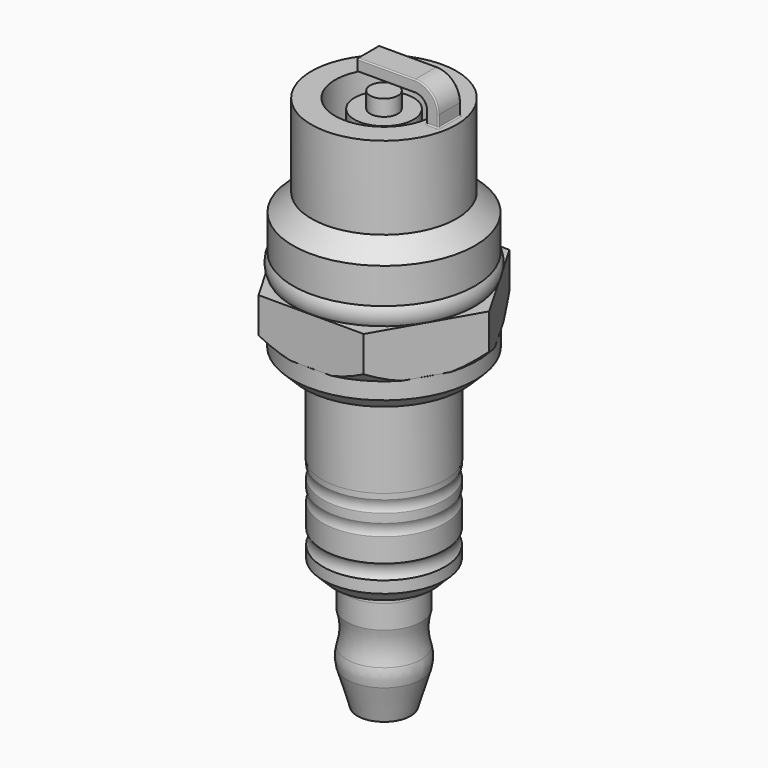
from build123d import *

# Parameters (mm, degrees)
F3_DEPTH  = 4
F4_R      = 2.5
F4_R_2    = 1.175
F5_DEPTH  = 4
F6_DEPTH  = 5.35
F7_SIZE   = 1
F11_DEPTH = 1.175
F12_R     = 1
F13_R     = 2
F14_R     = 0.1
F15_R     = 0.5


with BuildPart() as f1:
    # F0 (on Front) → F1 (revolve)
    with BuildSketch(Plane.XZ):
        with BuildLine():
            Line((4.136, 17.85), (0, 17.85))
            Line((0, 17.85), (0, -22.65))
            Line((0, -22.65), (2.25, -22.65))
            Line((2.25, -22.65), (3.15, -19.65))
            ThreePointArc((3.15, -19.65), (3.2600766272, -18.9), (3.15, -18.15))
            ThreePointArc((3.15, -18.15), (2.9445236292, -16.75), (3.15, -15.35))
            Line((3.15, -15.35), (3.15, -13.35))
            Line((3.15, -13.35), (3.175, -13.35))
            Line((3.175, -13.35), (3.175, -12.6))
            Line((3.175, -12.6), (5.15, -12.6))
            Line((5.15, -12.6), (5.15, -10.6))
            ThreePointArc((5.15, -10.6), (4.9551933495, -9.975), (5.15, -9.35))
            Line((5.15, -9.35), (5.15, -7.35))
            ThreePointArc((5.15, -7.35), (5.0297958971, -6.85), (5.15, -6.35))
            Line((5.15, -6.35), (5.15, -5.6))
            ThreePointArc((5.15, -5.6), (5.0297958971, -5.1), (5.15, -4.6))
            Line((5.15, -4.6), (5.15, -4.1))
            Line((5.15, -4.1), (5.2, -4.1))
            Line((5.2, -4.1), (5.2, 3.15))
            Line((5.2, 3.15), (7.725, 3.15))
            Line((7.725, 3.15), (7.725, 5.65))
            Line((7.725, 5.65), (8.9, 5.65))
            Line((8.9, 5.65), (8.9, 9.65))
            Line((8.9, 9.65), (7.7, 9.65))
            ThreePointArc((7.7, 9.65), (7.9009618943, 10.4), (7.7, 11.15))
            Line((7.7, 11.15), (7.7, 14.15))
            Line((7.7, 14.15), (6.136, 15.65))
            Line((6.136, 15.65), (6.136, 22.65))
            Line((6.136, 22.65), (4.136, 22.65))
            Line((4.136, 22.65), (4.136, 17.85))
        make_face()
    revolve(axis=Axis((0, 0, 0), (0, 0, -1)))

    # F2 (on face) → F3 (cut, through all)
    with BuildSketch(Plane.XY.offset(9.65)):
        with BuildLine():
            Line((-8.9, 0), (-4.45, 7.7076260937))
            ThreePointArc((-4.45, 7.7076260937), (-7.7076260937, 4.45), (-8.9, 0))
        make_face()
        with BuildLine():
            Line((-4.45, -7.7076260937), (-8.9, 0))
            ThreePointArc((-8.9, 0), (-7.7076260937, -4.45), (-4.45, -7.7076260937))
        make_face()
        with BuildLine():
            Line((4.45, -7.7076260937), (-4.45, -7.7076260937))
            ThreePointArc((-4.45, -7.7076260937), (0, -8.9), (4.45, -7.7076260937))
        make_face()
        with BuildLine():
            ThreePointArc((4.45, -7.7076260937), (7.7076260937, -4.45), (8.9, 0))
            Line((8.9, 0), (4.45, -7.7076260937))
        make_face()
        with BuildLine():
            ThreePointArc((8.9, 0), (7.7076260937, 4.45), (4.45, 7.7076260937))
            Line((4.45, 7.7076260937), (8.9, 0))
        make_face()
        with BuildLine():
            ThreePointArc((4.45, 7.7076260937), (0, 8.9), (-4.45, 7.7076260937))
            Line((-4.45, 7.7076260937), (4.45, 7.7076260937))
        make_face()
    extrude(amount=-F3_DEPTH, mode=Mode.SUBTRACT)

    # F4 (on face) → F5 (join)
    with BuildSketch(Plane.XY.offset(17.85)):
        Circle(F4_R)
        Circle(F4_R_2, mode=Mode.SUBTRACT)
    extrude(amount=F5_DEPTH)

    # F6 (add): a face of the model
    f6_faces = [f1.faces().sort_by_distance(p)[0] for p in [
        (0, 0, 17.85),
    ]]
    extrude(f6_faces, amount=F6_DEPTH)

    # F7
    f7_edges = [f1.edges().sort_by_distance(p)[0] for p in [
        (-7.725, 0, 3.15),
        (-5.15, 0, -12.6),
    ]]
    chamfer(f7_edges, length=F7_SIZE)

    # F8 (on Front) → F9 (revolve, cut)
    with BuildSketch(Plane.XZ):
        Polygon((7.9, 5.65), (8.9, 5.65), (8.9, 6.6499999995), align=None)
    revolve(axis=Axis((0, 0, 0), (0, 0, -1)), mode=Mode.SUBTRACT)

    # F10 (on Front) → F11 (join, symmetric)
    with BuildSketch(Plane.XZ):
        Polygon((5.536, 25.65), (-1.364, 25.65), (-1.364, 24.65), (4.536, 24.65), (4.536, 22.65), (5.536, 22.65), align=None)
    extrude(amount=F11_DEPTH, both=True)

    # F12
    f12_edges = [f1.edges().sort_by_distance(p)[0] for p in [
        (4.536, 0, 24.65),
    ]]
    fillet(f12_edges, radius=F12_R)

    # F13
    f13_edges = [f1.edges().sort_by_distance(p)[0] for p in [
        (5.536, 0, 25.65),
    ]]
    fillet(f13_edges, radius=F13_R)

    # F14
    f14_edges = [f1.edges().sort_by_distance(p)[0] for p in [
        (1.086, -1.175, 25.65),
        (4.950214, -1.175, 25.064214),
        (-1.364, -1.175, 25.15),
        (5.536, -1.175, 23.15),
        (1.086, -1.175, 24.65),
        (5.036, -1.175, 22.65),
        (4.243107, -1.175, 24.357107),
        (4.536, -1.175, 23.15),
        (-1.364, 0, 25.65),
        (-1.364, 1.175, 25.15),
        (-1.364, 0, 24.65),
        (1.086, 1.175, 25.65),
        (4.950214, 1.175, 25.064214),
        (5.536, 1.175, 23.15),
        (1.086, 1.175, 24.65),
        (5.036, 1.175, 22.65),
        (4.243107, 1.175, 24.357107),
        (4.536, 1.175, 23.15),
        (5.536, 0, 22.65),
        (4.536, 0, 22.65),
    ]]
    fillet(f14_edges, radius=F14_R)

    # F15
    f15_edges = [f1.edges().sort_by_distance(p)[0] for p in [
        (-5.2, 0, 3.15),
        (-3.175, 0, -12.6),
    ]]
    fillet(f15_edges, radius=F15_R)


solid = f1.part
